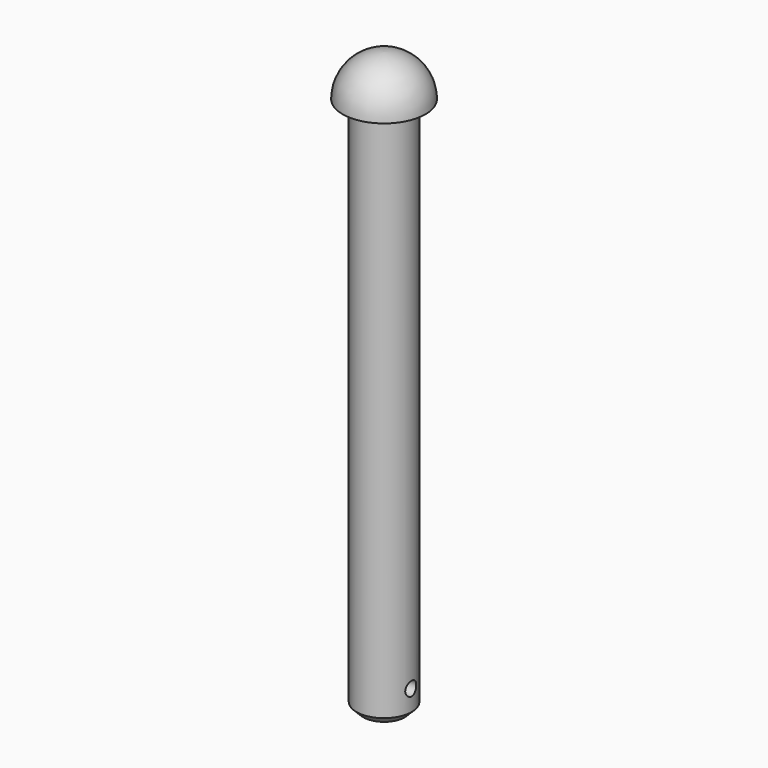
from build123d import *

# Parameters (mm, degrees)
F0_R     = 2
F1_DEPTH = 39
F2_SIZE2 = 0.5
F2_SIZE  = 0.5
F3_R     = 3
F4_DEPTH = 3
F5_R     = 2.99999
F6_R     = 0.5
F7_DEPTH = 12.5


# Not quite as in the source:
# - a fillet or chamfer is up to 0.001 mm smaller than in the source, because OpenCascade refuses the exact size


with BuildPart() as f1:
    # F0 (on Top) → F1 (new body)
    with BuildSketch(Plane.XY):
        Circle(F0_R)
    extrude(amount=F1_DEPTH)

    # F2
    f2_edges = [f1.edges().sort_by_distance(p)[0] for p in [
        (-2, 0, 0),
    ]]
    chamfer(f2_edges, length=F2_SIZE, length2=F2_SIZE2)

    # F3 (on face) → F4 (join)
    with BuildSketch(Plane.XY.offset(39)):
        Circle(F3_R)
    extrude(amount=F4_DEPTH)

    # F5 (radius 3 in the source; OpenCascade refuses exactly that, so slightly less here)
    f5_edges = [f1.edges().sort_by_distance(p)[0] for p in [
        (-3, 0, 42),
    ]]
    fillet(f5_edges, radius=F5_R)

    # F6 (on Right) → F7 (cut, symmetric)
    with BuildSketch(Plane.YZ):
        with Locations((0, 2)):
            Circle(F6_R)
    extrude(amount=F7_DEPTH, both=True, mode=Mode.SUBTRACT)


solid = f1.part
